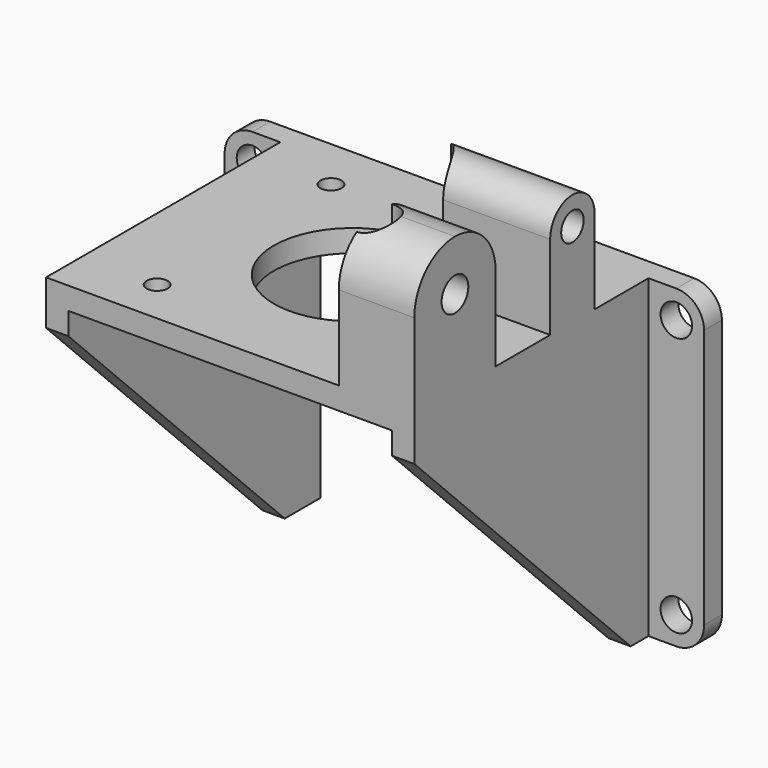
from build123d import *

# Parameters (mm, degrees)
F0_W         = 52.5309846
F0_H         = 44.9404867
F0_R         = 1.5
F0_R_2       = 11.2530001
F1_DEPTH     = 3.175
F2_W         = 3.175
F2_H         = 44.9404867
F3_DEPTH     = 41.774999
F4_W         = 7.9375
F4_H         = 3.175
F5_DEPTH     = 44.949999
F6_R         = 3.96875
F7_R         = 2.2479
F8_DEPTH     = 3.175
F10_DEPTH    = 52.5309846
F12_DEPTH    = 19.2659
F14_DEPTH    = 10.7654979
F15_T1_DEPTH = 47.0239979
F16_R        = 2
F17_DEPTH    = 134
F18_R        = 7.9375
F19_DEPTH    = 25.4


# Not quite as in the source:
# - a fillet or chamfer that OpenCascade refuses, or shapes differently, is made with other operations: its cross-section is extruded or revolved along the edge and cut away or added
# - an extrude ends at something that could not be found from the text; its depth is read off the source's solid
# - a feature names something its author has since deleted; it is built from what else it names


with BuildPart() as f1:
    # F0 (on Top) → F1 (new body)
    with BuildSketch(Plane.XY):
        with Locations((26.2654923, -22.47024335)):
            Rectangle(F0_W, F0_H)
        with Locations((10.7654979, -38.5904867)):
            Circle(F0_R, mode=Mode.SUBTRACT)
        with Locations((26.2654923, -23.0904923)):
            Circle(F0_R_2, mode=Mode.SUBTRACT)
        with Locations((41.7654867, -38.5904867)):
            Circle(F0_R, mode=Mode.SUBTRACT)
        with Locations((10.7654979, -7.5904979)):
            Circle(F0_R, mode=Mode.SUBTRACT)
        with Locations((41.7654867, -7.5904979)):
            Circle(F0_R, mode=Mode.SUBTRACT)
    extrude(amount=F1_DEPTH)

    # F2 (on face) → F3 (join)
    with BuildSketch(Plane(origin=(0, 0, 0), x_dir=(1, 0, 0), z_dir=(0, 0, -1))):
        with Locations((1.5875, 22.47024335)):
            Rectangle(F2_W, F2_H)
        with Locations((50.9434846, 22.47024335)):
            Rectangle(F2_W, F2_H)
    extrude(amount=F3_DEPTH)

    # F4 (on face) → F5 (join, through all)
    with BuildSketch(Plane(origin=(0, 0, -41.774999), x_dir=(1, 0, 0), z_dir=(0, 0, -1))):
        with Locations((-3.96875, 1.5875)):
            Rectangle(F4_W, F4_H)
        with Locations((56.4997346, 1.5875)):
            Rectangle(F4_W, F4_H)
    extrude(amount=-F5_DEPTH)

    # F6
    f6_edges = [f1.edges().sort_by_distance(p)[0] for p in [
        (60.468485, -1.5875, -41.774999),
        (60.468485, -1.5875, 3.175),
        (-7.9375, -1.5875, 3.175),
        (-7.9375, -1.5875, -41.774999),
    ]]
    fillet(f6_edges, radius=F6_R)

    # F7 (on face) → F8 (cut, through all)
    with BuildSketch(Plane(origin=(0, 0, 0), x_dir=(-1, 0, 0), z_dir=(0, 1, 0))):
        with Locations((3.96875, -37.806249)):
            Circle(F7_R)
        with Locations((3.96875, -0.79375)):
            Circle(F7_R)
        with Locations((-56.4997346, -0.79375)):
            Circle(F7_R)
        with Locations((-56.4997346, -37.806249)):
            Circle(F7_R)
    extrude(amount=-F8_DEPTH, mode=Mode.SUBTRACT)

    # F9 (on face) → F10 (cut, through all)
    with BuildSketch(Plane.YZ.offset(52.5309846)):
        Polygon((-44.9404867, -3.175), (-44.9404867, -41.774999), (-6.35, -41.774999), align=None)
    extrude(amount=-F10_DEPTH, mode=Mode.SUBTRACT)

    # F11 (on face) → F12 (join)
    with BuildSketch(Plane.XY.offset(3.175)):
        with BuildLine():
            Line((41.7654867, -44.9404867), (52.5309846, -44.9404867))
            Line((52.5309846, -44.9404867), (52.5309846, -30.4370867))
            Line((52.5309846, -30.4370867), (41.7654867, -30.4370867))
            Line((41.7654867, -30.4370867), (41.7654867, -35.4154867))
            ThreePointArc((41.7654867, -35.4154867), (44.9404867, -38.5904867), (41.7654867, -41.7654867))
            Line((41.7654867, -41.7654867), (41.7654867, -44.9404867))
        make_face()
        with BuildLine():
            Line((52.5309846, -20.7092423), (52.5309846, -12.7717423))
            Line((52.5309846, -12.7717423), (30.7547472146, -12.7717423))
            ThreePointArc((30.7547472146, -12.7717423), (34.966988133, -15.9550889113), (37.2636584966, -20.7092423))
            Line((37.2636584966, -20.7092423), (52.5309846, -20.7092423))
        make_face()
    extrude(amount=F12_DEPTH)

    # F13 (on face) → F14 (cut, through all)
    with BuildSketch(Plane.YZ.offset(52.5309846)):
        with BuildLine():
            Line((-40.0700367, 15.1892), (-37.6887867, 15.1892))
            Line((-37.6887867, 15.1892), (-37.6887867, 12.80795))
            ThreePointArc((-37.6887867, 12.80795), (-36.0049886773, 13.5054019773), (-35.3075367, 15.1892))
            ThreePointArc((-35.3075367, 15.1892), (-37.6887867, 17.57045), (-40.0700367, 15.1892))
        make_face()
        with BuildLine():
            Line((-37.6887867, 12.80795), (-37.6887867, 15.1892))
            Line((-37.6887867, 15.1892), (-40.0700367, 15.1892))
            ThreePointArc((-40.0700367, 15.1892), (-39.3725847227, 13.5054019773), (-37.6887867, 12.80795))
        make_face()
    extrude(amount=-F14_DEPTH, mode=Mode.SUBTRACT)

    # F15: fillet of radius 7.2517 on 2 edges, made by hand

    # F15_s2 → F15_t1 (cut)
    with BuildSketch(Plane.YZ.offset(23.6362367)):
        with BuildLine():
            ThreePointArc((-44.9404867, 15.1892), (-42.8165129451, 20.3169262451), (-37.6887867, 22.4409))
            Line((-37.6887867, 22.4409), (-44.9404867, 22.4409))
            Line((-44.9404867, 22.4409), (-44.9404867, 15.1892))
        make_face()
        with BuildLine():
            ThreePointArc((-30.4370867, 15.1892), (-32.5610604549, 20.3169262451), (-37.6887867, 22.4409))
            Line((-37.6887867, 22.4409), (-30.4370867, 22.4409))
            Line((-30.4370867, 22.4409), (-30.4370867, 15.1892))
        make_face()
    extrude(amount=F15_T1_DEPTH, mode=Mode.SUBTRACT)

    # F16 (on face) → F17 (cut, through all)
    with BuildSketch(Plane.YZ.offset(52.5309846)):
        with BuildLine():
            Line((-12.7717423, 22.4409), (-20.7092423, 22.4409))
            Line((-20.7092423, 22.4409), (-20.7092423, 15.1892))
            ThreePointArc((-20.7092423, 15.1892), (-16.7404923, 19.15795), (-12.7717423, 15.1892))
            Line((-12.7717423, 15.1892), (-12.7717423, 22.4409))
        make_face()
        with Locations((-16.7404923, 15.1892)):
            Circle(F16_R)
    extrude(amount=-F17_DEPTH, mode=Mode.SUBTRACT)

    # F18 (on face) → F19 (cut)
    with BuildSketch(Plane.XY.offset(3.175)):
        with Locations((26.2654923, -10.3904923)):
            Circle(F18_R)
    extrude(amount=F19_DEPTH, mode=Mode.SUBTRACT)


solid = f1.part
